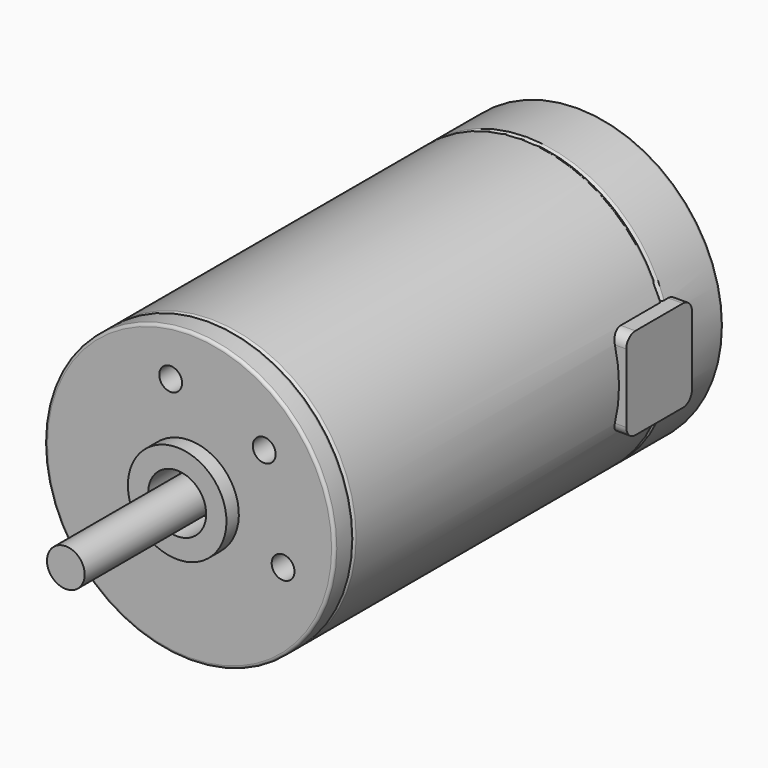
from build123d import *

# Parameters (mm, degrees)
F0_W     = 23.495
F0_H     = 2.4765
F2_DEPTH = 20
F3_R     = 1.5
F4_DEPTH = 5


# Not quite as in the source:
# - a feature names something its author has since deleted; it is built from what else it names


with BuildPart() as f1:
    # F0 (on Right) → F1 (revolve)
    with BuildSketch(Plane.YZ):
        with Locations((11.7475, 1.23825)):
            Rectangle(F0_W, F0_H)
        with BuildLine():
            Line((23.114, 19.05), (20.701, 19.05))
            ThreePointArc((20.701, 19.05), (20.4315923164, 18.9384076836), (20.32, 18.669))
            Line((20.32, 18.669), (20.32, 6.477))
            Line((20.32, 6.477), (18.288, 6.477))
            Line((18.288, 6.477), (18.288, 3.81))
            Line((18.288, 3.81), (23.495, 3.81))
            Line((23.495, 3.81), (23.495, 18.669))
            ThreePointArc((23.495, 18.669), (23.3834076836, 18.9384076836), (23.114, 19.05))
        make_face()
        with BuildLine():
            Line((76.351, 6.0325), (75.311, 6.0325))
            Line((75.311, 6.0325), (75.311, 0))
            Line((75.311, 0), (77.851, 0))
            Line((77.851, 0), (77.851, 4.5325))
            ThreePointArc((77.851, 4.5325), (77.4116601718, 5.5931601718), (76.351, 6.0325))
        make_face()
        with BuildLine():
            Line((67.056, 4.5325), (67.056, 0))
            Line((67.056, 0), (75.311, 0))
            Line((75.311, 0), (75.311, 6.0325))
            Line((75.311, 6.0325), (68.556, 6.0325))
            ThreePointArc((68.556, 6.0325), (67.4953398282, 5.5931601718), (67.056, 4.5325))
        make_face()
        with BuildLine():
            ThreePointArc((75.692, 19.05), (75.4225923164, 18.9384076836), (75.311, 18.669))
            Line((75.311, 18.669), (75.311, 6.0325))
            Line((75.311, 6.0325), (76.351, 6.0325))
            ThreePointArc((76.351, 6.0325), (77.4116601718, 5.5931601718), (77.851, 4.5325))
            Line((77.851, 4.5325), (77.851, 0))
            Line((77.851, 0), (84.201, 0))
            Line((84.201, 0), (84.201, 18.669))
            ThreePointArc((84.201, 18.669), (84.0894076836, 18.9384076836), (83.82, 19.05))
            Line((83.82, 19.05), (75.692, 19.05))
        make_face()
        with BuildLine():
            ThreePointArc((23.876, 19.05), (23.6065923164, 18.9384076836), (23.495, 18.669))
            Line((23.495, 18.669), (23.495, 3.81))
            Line((23.495, 3.81), (23.495, 2.4765))
            Line((23.495, 2.4765), (23.495, 0))
            Line((23.495, 0), (67.056, 0))
            Line((67.056, 0), (67.056, 4.5325))
            ThreePointArc((67.056, 4.5325), (67.4953398282, 5.5931601718), (68.556, 6.0325))
            Line((68.556, 6.0325), (75.311, 6.0325))
            Line((75.311, 6.0325), (75.311, 18.669))
            ThreePointArc((75.311, 18.669), (75.1994076836, 18.9384076836), (74.93, 19.05))
            Line((74.93, 19.05), (23.876, 19.05))
        make_face()
    revolve(axis=Axis((0, 11.7475, 0), (0, 1, 0)))

    # F0 (on Right) → F2 (join)
    with BuildSketch(Plane.YZ):
        with BuildLine():
            Line((76.351, 6.0325), (75.311, 6.0325))
            Line((75.311, 6.0325), (75.311, 0))
            Line((75.311, 0), (77.851, 0))
            Line((77.851, 0), (77.851, 4.5325))
            ThreePointArc((77.851, 4.5325), (77.4116601718, 5.5931601718), (76.351, 6.0325))
        make_face()
        with BuildLine():
            Line((75.311, 0), (67.056, 0))
            Line((67.056, 0), (67.056, -4.5325))
            ThreePointArc((67.056, -4.5325), (67.4953398282, -5.5931601718), (68.556, -6.0325))
            Line((68.556, -6.0325), (76.351, -6.0325))
            ThreePointArc((76.351, -6.0325), (77.4116601718, -5.5931601718), (77.851, -4.5325))
            Line((77.851, -4.5325), (77.851, 0))
            Line((77.851, 0), (75.311, 0))
        make_face()
        with BuildLine():
            Line((67.056, 4.5325), (67.056, 0))
            Line((67.056, 0), (75.311, 0))
            Line((75.311, 0), (75.311, 6.0325))
            Line((75.311, 6.0325), (68.556, 6.0325))
            ThreePointArc((68.556, 6.0325), (67.4953398282, 5.5931601718), (67.056, 4.5325))
        make_face()
    extrude(amount=F2_DEPTH)

    # F3 (on face) → F4 (cut)
    with BuildSketch(Plane.XZ.offset(-20.32)):
        with Locations((-9.8112245429, -8.5287673769)):
            Circle(F3_R)
        with Locations((-2.4805169399, 12.7611533848)):
            Circle(F3_R)
        with Locations((9.8112245429, 8.5287673769)):
            Circle(F3_R)
        with Locations((12.2917414828, -4.2323860079)):
            Circle(F3_R)
    extrude(amount=-F4_DEPTH, mode=Mode.SUBTRACT)


solid = f1.part
